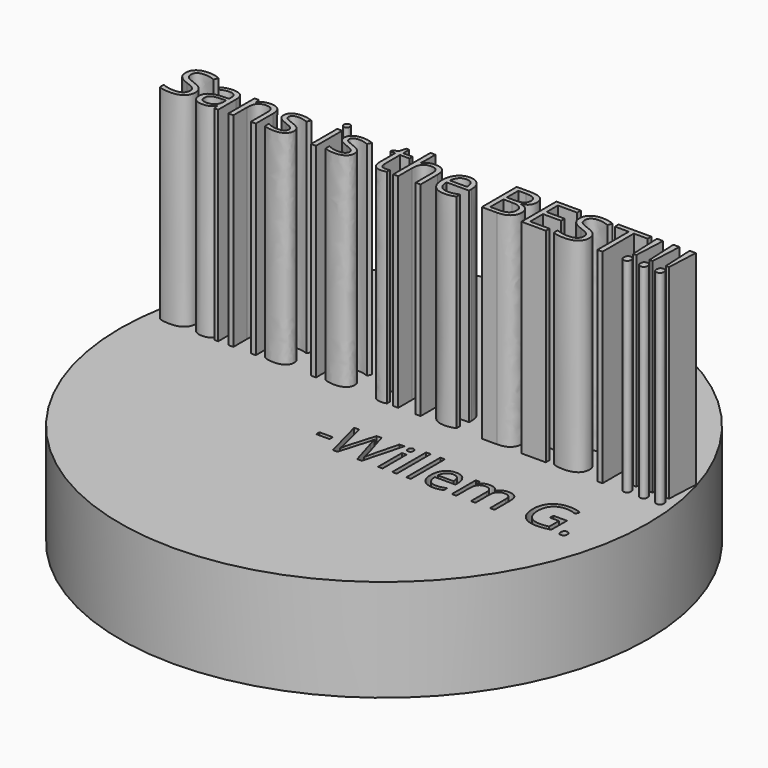
from build123d import *

# Parameters (mm, degrees)
F0_R         = 65.7573040502
F0_R_2       = 57.9371930215
F0_R_3       = 50.9142988695
F0_R_4       = 43.7425725946
F1_DEPTH     = 25.4
F2_TEXT_SIZE = 15.245812466
F3_DEPTH     = 50.8
F4_TEXT_SIZE = 13.9284749619
F5_DEPTH     = 25.4
F6_W         = 3.3384813424
F6_H         = 1.0337540011
F6_W_2       = 1.1295122664
F6_H_2       = 7.4539104288
F6_H_3       = 10.5834646468
F7_DEPTH     = 25.4


# Not quite as in the source:
# - Text() gives the source's letters only with a copy of the font that has no kerning and outlines rounded to 1/6400 em; it was checked with that copy


with BuildPart() as f1:
    # F0 (on Top) → F1 (new body)
    with BuildSketch(Plane.XY):
        Circle(F0_R)
        Circle(F0_R_2, mode=Mode.SUBTRACT)
        Circle(F0_R_2)
        Circle(F0_R_3, mode=Mode.SUBTRACT)
        Circle(F0_R_3)
        Circle(F0_R_4, mode=Mode.SUBTRACT)
        Circle(F0_R_4)
        Polygon((-10.0285010412, -12.6446327195), (-31.6115804017, 3.70618538), (-10.0285010412, 3.70618538), (0, 27.9053952545), (11.772589758, 3.70618538), (32.7016338706, 3.70618538), (11.772589758, -12.6446327195), (19.6209810674, -28.3414162695), (0, -12.6446327195), (-12.557425797, -28.3414162695), align=None, mode=Mode.SUBTRACT)
        Polygon((-10.0285010412, 3.70618538), (-31.6115804017, 3.70618538), (-10.0285010412, -12.6446327195), (-12.557425797, -28.3414162695), (0, -12.6446327195), (19.6209810674, -28.3414162695), (11.772589758, -12.6446327195), (32.7016338706, 3.70618538), (11.772589758, 3.70618538), (0, 27.9053952545), align=None)
    extrude(amount=F1_DEPTH)

    # F2 (on face) → F3 (join)
    with BuildSketch(Plane.XY.offset(25.4)):
        with Locations((-63.05720884, 7.6727187556)):
            Text('Sans is the BEST!!!', F2_TEXT_SIZE, font='Open Sans', text_align=(TextAlign.LEFT, TextAlign.BOTTOM))
    extrude(amount=F3_DEPTH)

    # F4 (on face) → F5 (cut)
    with BuildSketch(Plane.XY.offset(25.4)):
        with Locations((-8.7204352021, -14.1707086004)):
            Text('-Willem G.', F4_TEXT_SIZE, font='Open Sans', text_align=(TextAlign.LEFT, TextAlign.BOTTOM))
    extrude(amount=-F5_DEPTH, mode=Mode.SUBTRACT)

    # F6 (on face) → F7 (cut)
    with BuildSketch(Plane(origin=(0, 0, 0), x_dir=(1, 0, 0), z_dir=(0, 0, -1))):
        with Locations((-6.4788212629, 10.4372244134)):
            Rectangle(F6_W, F6_H)
        with BuildLine():
            Line((5.8065289183, 14.1707086004), (4.6639587066, 14.1707086004))
            Line((4.6639587066, 14.1707086004), (2.6573877824, 7.5133328335))
            add(Edge.make_bspline(
                [(2.1546568892, 5.5872859052), (2.1611858618, 5.7243943306), (2.5137503843, 7.0693626941), (2.6573877824, 7.5133328335)],
                knots=[0, 0, 0, 1, 2, 2, 2], degree=2))
            add(Edge.make_bspline(
                [(2.1546568892, 5.5872859052), (2.0044905185, 6.4861078051), (1.6780418866, 7.5525066693)],
                knots=[0, 0, 0, 1, 1, 1], degree=2))
            Line((1.6780418866, 7.5525066693), (-0.2675919596, 14.1707086004))
            Line((-0.2675919596, 14.1707086004), (-1.4101621713, 14.1707086004))
            Line((-1.4101621713, 14.1707086004), (-4.0565724141, 4.2270832722))
            Line((-4.0565724141, 4.2270832722), (-2.8313018823, 4.2270832722))
            Line((-2.8313018823, 4.2270832722), (-1.2599958007, 10.3686702007))
            add(Edge.make_bspline(
                [(-1.2599958007, 10.3686702007), (-0.9335471687, 11.6614067831), (-0.7833807981, 12.7082187294)],
                knots=[0, 0, 0, 1, 1, 1], degree=2))
            add(Edge.make_bspline(
                [(-0.7833807981, 12.7082187294), (-0.6005695642, 11.4633612797), (-0.2392997449, 10.2729119353)],
                knots=[0, 0, 0, 1, 1, 1], degree=2))
            Line((-0.2392997449, 10.2729119353), (1.5409334612, 4.2270832722))
            Line((1.5409334612, 4.2270832722), (2.766203993, 4.2270832722))
            Line((2.766203993, 4.2270832722), (4.6356664918, 10.3273200406))
            add(Edge.make_bspline(
                [(4.6356664918, 10.3273200406), (4.9621151237, 11.3828372838), (5.1862765176, 12.7082187294)],
                knots=[0, 0, 0, 1, 1, 1], degree=2))
            add(Edge.make_bspline(
                [(5.1862765176, 12.7082187294), (5.3168559704, 11.741930779), (5.6759494655, 10.3556122554)],
                knots=[0, 0, 0, 1, 1, 1], degree=2))
            Line((5.6759494655, 10.3556122554), (7.2407265745, 4.2270832722))
            Line((7.2407265745, 4.2270832722), (8.4659971063, 4.2270832722))
            Line((8.4659971063, 4.2270832722), (5.8065289183, 14.1707086004))
        make_face()
        with Locations((10.4170717631, 10.443753386)):
            Rectangle(F6_W_2, F6_H_2)
        with BuildLine():
            add(Edge.make_bspline(
                [(54.7890579756, 13.450345286), (54.7890579756, 13.9400182339), (55.2439097361, 14.3687541038), (55.97950732, 14.3687541038), (56.4278301079, 13.8921391012), (56.4278301079, 12.9933172013), (55.9860362927, 12.5254074956), (55.2047359003, 12.5254074956), (54.7890579756, 12.9933172013), (54.7890579756, 13.450345286)],
                knots=[0, 0, 0, 1, 2, 3.1125, 4.225, 5.375862069, 6.5267241379, 7.658511145, 8.790298152, 8.790298152, 8.790298152], degree=2))
        make_face()
        with BuildLine():
            Line((37.7397340926, 14.1707086004), (37.7397340926, 9.3218582543))
            add(Edge.make_bspline(
                [(34.1139779541, 10.0074003814), (34.1139779541, 8.7494849864), (35.1216160646, 7.539448724), (36.9780206181, 7.539448724), (37.7397340926, 8.4295653271), (37.7397340926, 9.3218582543)],
                knots=[0, 0, 0, 1, 2, 2.7623966942, 3.5247933884, 3.5247933884, 3.5247933884], degree=2))
            Line((34.1139779541, 10.0074003814), (34.1139779541, 14.1707086004))
            Line((34.1139779541, 14.1707086004), (32.9844656877, 14.1707086004))
            Line((32.9844656877, 14.1707086004), (32.9844656877, 9.3218582543))
            add(Edge.make_bspline(
                [(29.367414846, 10.25985399), (29.367414846, 8.8104220643), (30.3532897144, 7.539448724), (32.2227522132, 7.539448724), (32.9844656877, 8.4295653271), (32.9844656877, 9.3218582543)],
                knots=[0, 0, 0, 1, 2, 2.7638603696, 3.5277207392, 3.5277207392, 3.5277207392], degree=2))
            Line((29.367414846, 10.25985399), (29.367414846, 14.1707086004))
            Line((29.367414846, 14.1707086004), (28.2379025796, 14.1707086004))
            Line((28.2379025796, 14.1707086004), (28.2379025796, 6.7167981716))
            Line((28.2379025796, 6.7167981716), (29.1563113974, 6.7167981716))
            Line((29.1563113974, 6.7167981716), (29.3391226312, 7.7374942274))
            Line((29.3391226312, 7.7374942274), (29.3935307365, 7.7374942274))
            add(Edge.make_bspline(
                [(33.8832875875, 7.8463104381), (33.345735507, 6.5796897462), (30.8777838497, 6.5796897462), (29.7134503958, 7.1934131742), (29.3935307365, 7.7374942274)],
                knots=[0, 0, 0, 1, 1.4122042341, 1.8244084682, 1.8244084682, 1.8244084682], degree=2))
            Line((33.8832875875, 7.8463104381), (33.9376956929, 7.8463104381))
            add(Edge.make_bspline(
                [(38.8670700348, 9.308800309), (38.8670700348, 7.8789553012), (37.6091546398, 6.5796897462), (35.5351176651, 6.5796897462), (34.2706732974, 7.2608792248), (33.9376956929, 7.8463104381)],
                knots=[0, 0, 0, 1, 2, 2.6402753873, 3.2805507745, 3.2805507745, 3.2805507745], degree=2))
            Line((38.8670700348, 9.308800309), (38.8670700348, 14.1707086004))
            Line((38.8670700348, 14.1707086004), (37.7397340926, 14.1707086004))
        make_face()
        with BuildLine():
            Line((49.3569527405, 8.960588435), (52.736784243, 8.960588435))
            Line((52.736784243, 8.960588435), (52.736784243, 13.7963808358))
            add(Edge.make_bspline(
                [(52.5866178723, 4.6688770874), (51.213357294, 4.0856221983), (48.0511582128, 4.0856221983), (45.7116096841, 5.3152453786), (44.4667522344, 7.6482649347), (44.4667522344, 11.620056623), (46.9825830243, 14.3078170258), (50.3145353941, 14.3078170258), (51.9467785537, 14.0488344445), (52.736784243, 13.7963808358)],
                knots=[0, 0, 0, 1, 1.9849726776, 2.9699453552, 3.9549180328, 5.4910886043, 7.0272591758, 7.7590511356, 8.4908430954, 8.4908430954, 8.4908430954], degree=2))
            Line((52.5866178723, 4.6688770874), (52.1382950845, 5.6895731432))
            add(Edge.make_bspline(
                [(51.5789797618, 13.0542542793), (50.5931048934, 13.2936499427), (47.6550672061, 13.2936499427), (45.6898464419, 11.2130839952), (45.6898464419, 7.2804661427), (47.7312385535, 5.1193761994), (50.7911503967, 5.1193761994), (52.1382950845, 5.6895731432)],
                knots=[0, 0, 0, 1, 2.8421052632, 4.6842105263, 6.4406827881, 8.1971550498, 9.4018338672, 9.4018338672, 9.4018338672], degree=2))
            Line((51.5789797618, 13.0542542793), (51.5789797618, 9.9943424361))
            Line((51.5789797618, 9.9943424361), (49.3569527405, 9.9943424361))
            Line((49.3569527405, 9.9943424361), (49.3569527405, 8.960588435))
        make_face()
        with Locations((13.9405406636, 8.878976277)):
            Rectangle(F6_W_2, F6_H_3)
        with Locations((17.4640095641, 8.878976277)):
            Rectangle(F6_W_2, F6_H_3)
        with BuildLine():
            add(Edge.make_bspline(
                [(9.7565573645, 4.6971693021), (9.7565573645, 5.0780260394), (10.1374141017, 5.452353804), (10.6967294244, 5.452353804), (11.0906441069, 5.0780260394), (11.0906441069, 4.3163125649), (10.6967294244, 3.9485137729), (10.1374141017, 3.9485137729), (9.7565573645, 4.3097835923), (9.7565573645, 4.6971693021)],
                knots=[0, 0, 0, 1, 2, 2.946969697, 3.8939393939, 4.8409090909, 5.7878787879, 6.7878787879, 7.7878787879, 7.7878787879, 7.7878787879], degree=2))
        make_face()
    extrude(amount=-F7_DEPTH, mode=Mode.SUBTRACT)


solid = f1.part
